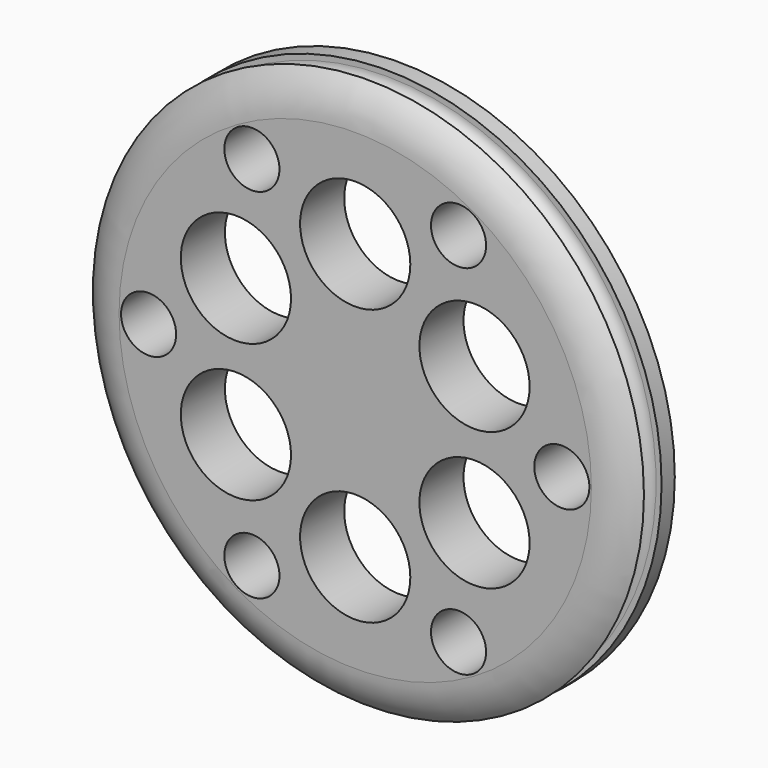
from build123d import *

# Parameters (mm, degrees)
F0_R     = 25
F0_R_2   = 2.5
F0_R_3   = 5
F1_DEPTH = 5


# Not quite as in the source:
# - a fillet or chamfer that OpenCascade refuses, or shapes differently, is made with other operations: its cross-section is extruded or revolved along the edge and cut away or added


with BuildPart() as f1:
    # F0 (on Front) → F1 (new body)
    with BuildSketch(Plane.XZ):
        Circle(F0_R)
        with Locations((-9.375, -16.237976321)):
            Circle(F0_R_2, mode=Mode.SUBTRACT)
        with Locations((-10.8253175473, -6.25)):
            Circle(F0_R_3, mode=Mode.SUBTRACT)
        with Locations((9.375, -16.237976321)):
            Circle(F0_R_2, mode=Mode.SUBTRACT)
        with Locations((0, -12.5)):
            Circle(F0_R_3, mode=Mode.SUBTRACT)
        with Locations((10.8253175473, -6.25)):
            Circle(F0_R_3, mode=Mode.SUBTRACT)
        with Locations((-18.75, 0)):
            Circle(F0_R_2, mode=Mode.SUBTRACT)
        with Locations((-10.8253175473, 6.25)):
            Circle(F0_R_3, mode=Mode.SUBTRACT)
        with Locations((-9.375, 16.237976321)):
            Circle(F0_R_2, mode=Mode.SUBTRACT)
        with Locations((10.8253175473, 6.25)):
            Circle(F0_R_3, mode=Mode.SUBTRACT)
        with Locations((18.75, 0)):
            Circle(F0_R_2, mode=Mode.SUBTRACT)
        with Locations((0, 12.5)):
            Circle(F0_R_3, mode=Mode.SUBTRACT)
        with Locations((9.375, 16.237976321)):
            Circle(F0_R_2, mode=Mode.SUBTRACT)
    extrude(amount=F1_DEPTH)

    # F3 (on Right) → F5 (revolve, cut)
    with BuildSketch(Plane.YZ):
        with BuildLine():
            Line((-3.5, 25), (-3.5, 24.5))
            ThreePointArc((-3.5, 24.5), (-3.4659258263, 24.7588190451), (-3.3660254038, 25))
            Line((-3.3660254038, 25), (-3.5, 25))
        make_face()
        with BuildLine():
            ThreePointArc((-3.3660254038, 25), (-3.4659258263, 24.7588190451), (-3.5, 24.5))
            ThreePointArc((-3.5, 24.5), (-2.5, 23.5), (-1.5, 24.5))
            ThreePointArc((-1.5, 24.5), (-1.5340741737, 24.7588190451), (-1.6339745962, 25))
            Line((-1.6339745962, 25), (-3.3660254038, 25))
        make_face()
        with BuildLine():
            ThreePointArc((-1.6339745962, 25), (-2.5, 25.5), (-3.3660254038, 25))
            Line((-3.3660254038, 25), (-1.6339745962, 25))
        make_face()
        with BuildLine():
            ThreePointArc((-1.6339745962, 25), (-1.5340741737, 24.7588190451), (-1.5, 24.5))
            Line((-1.5, 24.5), (-1.5, 25))
            Line((-1.5, 25), (-1.6339745962, 25))
        make_face()
    revolve(axis=Axis((0, -2.5, 0), (0, -1, 0)), mode=Mode.SUBTRACT)

    # F6: fillet of radius 5 on 1 edges, made by hand

    # F6_s1 → F6_t2 (revolve, cut)
    with BuildSketch(Plane.XY):
        with BuildLine():
            ThreePointArc((25, -3.5), (23.3657774588, -4.6097722286), (21.4292857857, -5))
            Line((21.4292857857, -5), (25, -5))
            Line((25, -5), (25, -3.5))
        make_face()
    revolve(axis=Axis((0, -5, 0), (0, -1, 0)), mode=Mode.SUBTRACT)


solid = f1.part
